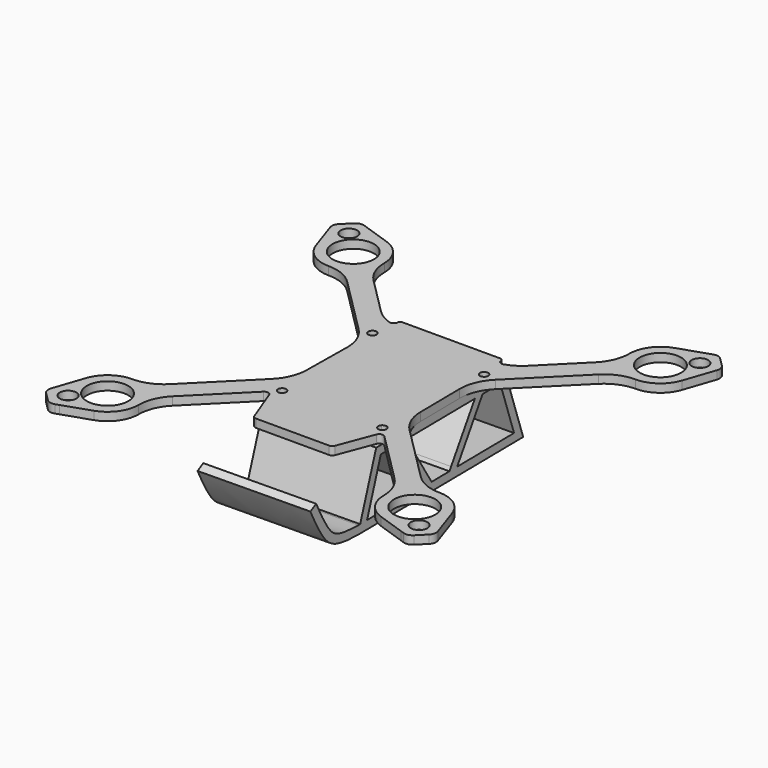
from build123d import *

# Parameters (mm, degrees)
F0_R     = 5
F0_R_2   = 1
F0_R_3   = 2
F1_DEPTH = 2
F3_DEPTH = 27


# Not quite as in the source:
# - the dataset's text gives a spline's control points without its knots; the knots are read off the source's solid


with BuildPart() as f1:
    # F0 (on Top) → F1 (new body)
    with BuildSketch(Plane.XY):
        with BuildLine():
            ThreePointArc((12.9701819491, -18.499116473), (13.6954441232, -17.876782257), (14.6119679801, -18.147501886))
            Line((14.6119679801, -18.147501886), (26.833136275, -30.3686701809))
            ThreePointArc((26.833136275, -30.3686701809), (28.8991826346, -33.4687011785), (29.6231060123, -37.1231060123))
            ThreePointArc((29.6231060123, -37.1231060123), (31.0266053165, -41.491478623), (34.7118204833, -44.2249157885))
            Line((34.7118204833, -44.2249157885), (41.2398543388, -46.4413865283))
            Line((41.2398543388, -46.4413865283), (42.1736187239, -46.7584286092))
            ThreePointArc((42.1736187239, -46.7584286092), (43.270713594, -46.8123822788), (44.2308417607, -46.2788262312))
            Line((44.2308417607, -46.2788262312), (46.2788262312, -44.2308417607))
            ThreePointArc((46.2788262312, -44.2308417607), (46.8123822788, -43.270713594), (46.7584286092, -42.1736187239))
            Line((46.7584286092, -42.1736187239), (44.2249157885, -34.7118204833))
            ThreePointArc((44.2249157885, -34.7118204833), (41.491478623, -31.0266053165), (37.1231060123, -29.6231060123))
            ThreePointArc((37.1231060123, -29.6231060123), (33.4687011785, -28.8991826346), (30.3686701809, -26.833136275))
            Line((30.3686701809, -26.833136275), (16.6740032779, -13.138469372))
            ThreePointArc((16.6740032779, -13.138469372), (14.5304846569, -9.9521662726), (13.7458594821, -6.1929691703))
            Line((13.7458594821, -6.1929691703), (13.595363536, 5.7913380039))
            ThreePointArc((13.595363536, 5.7913380039), (14.3319351196, 9.685658695), (16.5235073318, 12.9879734259))
            Line((16.5235073318, 12.9879734259), (30.3686701809, 26.833136275))
            ThreePointArc((30.3686701809, 26.833136275), (33.4687011785, 28.8991826346), (37.1231060123, 29.6231060123))
            ThreePointArc((37.1231060123, 29.6231060123), (41.491478623, 31.0266053165), (44.2249157885, 34.7118204833))
            Line((44.2249157885, 34.7118204833), (46.7584286092, 42.1736187239))
            ThreePointArc((46.7584286092, 42.1736187239), (46.8123822788, 43.270713594), (46.2788262312, 44.2308417607))
            Line((46.2788262312, 44.2308417607), (44.2308417607, 46.2788262312))
            ThreePointArc((44.2308417607, 46.2788262312), (43.270713594, 46.8123822788), (42.1736187239, 46.7584286092))
            Line((42.1736187239, 46.7584286092), (34.7118204833, 44.2249157885))
            ThreePointArc((34.7118204833, 44.2249157885), (31.0266053165, 41.491478623), (29.6231060123, 37.1231060123))
            ThreePointArc((29.6231060123, 37.1231060123), (28.8991826346, 33.4687011785), (26.833136275, 30.3686701809))
            Line((26.833136275, 30.3686701809), (17.7702922699, 21.3058261758))
            ThreePointArc((17.7702922699, 21.3058261758), (15.9339308633, 19.8564568598), (13.811079491, 18.8734020898))
            ThreePointArc((13.811079491, 18.8734020898), (12.9130317821, 19.0140644564), (12.4998939877, 19.8237512796))
            ThreePointArc((12.4998939877, 19.8237512796), (12.2538790329, 20.1992659281), (11.8415892299, 20.3768939877))
            Line((11.8415892299, 20.3768939877), (11.6629678581, 20.3768939877))
            Line((11.6629678581, 20.3768939877), (0, 20.3768939877))
            Line((0, 20.3768939877), (-11.6629678581, 20.3768939877))
            ThreePointArc((-11.6629678581, 20.3768939877), (-12.1822006328, 20.2527910691), (-12.4998939877, 19.8237512796))
            ThreePointArc((-12.4998939877, 19.8237512796), (-12.9130317821, 19.0140644564), (-13.811079491, 18.8734020898))
            ThreePointArc((-13.811079491, 18.8734020898), (-15.9339308633, 19.8564568598), (-17.7702922699, 21.3058261758))
            Line((-17.7702922699, 21.3058261758), (-26.833136275, 30.3686701809))
            ThreePointArc((-26.833136275, 30.3686701809), (-28.8991826346, 33.4687011785), (-29.6231060123, 37.1231060123))
            ThreePointArc((-29.6231060123, 37.1231060123), (-31.0266053165, 41.491478623), (-34.7118204833, 44.2249157885))
            Line((-34.7118204833, 44.2249157885), (-42.1736187239, 46.7584286092))
            ThreePointArc((-42.1736187239, 46.7584286092), (-43.270713594, 46.8123822788), (-44.2308417607, 46.2788262312))
            Line((-44.2308417607, 46.2788262312), (-46.2788262312, 44.2308417607))
            ThreePointArc((-46.2788262312, 44.2308417607), (-46.8123822788, 43.270713594), (-46.7584286092, 42.1736187239))
            Line((-46.7584286092, 42.1736187239), (-44.2249157885, 34.7118204833))
            ThreePointArc((-44.2249157885, 34.7118204833), (-41.491478623, 31.0266053165), (-37.1231060123, 29.6231060123))
            ThreePointArc((-37.1231060123, 29.6231060123), (-33.4687011785, 28.8991826346), (-30.3686701809, 26.833136275))
            Line((-30.3686701809, 26.833136275), (-16.5235073318, 12.9879734259))
            ThreePointArc((-16.5235073318, 12.9879734259), (-14.3319351196, 9.685658695), (-13.595363536, 5.7913380039))
            Line((-13.595363536, 5.7913380039), (-13.7458594821, -6.1929691703))
            ThreePointArc((-13.7458594821, -6.1929691703), (-14.5304846569, -9.9521662726), (-16.6740032779, -13.138469372))
            Line((-16.6740032779, -13.138469372), (-30.3686701809, -26.833136275))
            ThreePointArc((-30.3686701809, -26.833136275), (-33.4687011785, -28.8991826346), (-37.1231060123, -29.6231060123))
            ThreePointArc((-37.1231060123, -29.6231060123), (-41.491478623, -31.0266053165), (-44.2249157885, -34.7118204833))
            Line((-44.2249157885, -34.7118204833), (-46.7584286092, -42.1736187239))
            ThreePointArc((-46.7584286092, -42.1736187239), (-46.8123822788, -43.270713594), (-46.2788262312, -44.2308417607))
            Line((-46.2788262312, -44.2308417607), (-44.2308417607, -46.2788262312))
            ThreePointArc((-44.2308417607, -46.2788262312), (-43.270713594, -46.8123822788), (-42.1736187239, -46.7584286092))
            Line((-42.1736187239, -46.7584286092), (-41.2398543388, -46.4413865283))
            Line((-41.2398543388, -46.4413865283), (-34.7118204833, -44.2249157885))
            ThreePointArc((-34.7118204833, -44.2249157885), (-31.0266053165, -41.491478623), (-29.6231060123, -37.1231060123))
            ThreePointArc((-29.6231060123, -37.1231060123), (-28.8991826346, -33.4687011785), (-26.833136275, -30.3686701809))
            Line((-26.833136275, -30.3686701809), (-14.6119679801, -18.147501886))
            ThreePointArc((-14.6119679801, -18.147501886), (-13.6954441232, -17.876782257), (-12.9701819491, -18.499116473))
            Line((-12.9701819491, -18.499116473), (-9.7451295395, -26.9785982064))
            ThreePointArc((-9.7451295395, -26.9785982064), (-9.3781244066, -27.4463593737), (-8.8104502897, -27.6231060123))
            Line((-8.8104502897, -27.6231060123), (0, -27.6231060123))
            Line((0, -27.6231060123), (8.8104502897, -27.6231060123))
            ThreePointArc((8.8104502897, -27.6231060123), (9.3781244066, -27.4463593737), (9.7451295395, -26.9785982064))
            Line((9.7451295395, -26.9785982064), (12.9701819491, -18.499116473))
        make_face()
        with BuildLine():
            ThreePointArc((-40.4264068712, -42.4264068712), (-41.6610400065, -44.2741659362), (-43.8406204336, -43.8406204336))
            ThreePointArc((-43.8406204336, -43.8406204336), (-43.1917737359, -40.5786478062), (-40.4264068712, -42.4264068712))
        make_face(mode=Mode.SUBTRACT)
        with Locations((-37.1231060123, -37.1231060123)):
            Circle(F0_R, mode=Mode.SUBTRACT)
        with Locations((-12.1231060123, -15.6231060123)):
            Circle(F0_R_2, mode=Mode.SUBTRACT)
        with BuildLine():
            ThreePointArc((44.4264068712, -42.4264068712), (44.2741659362, -43.1917737359), (43.8406204336, -43.8406204336))
            ThreePointArc((43.8406204336, -43.8406204336), (40.5786478062, -41.6610400065), (44.4264068712, -42.4264068712))
        make_face(mode=Mode.SUBTRACT)
        with Locations((37.1231060123, -37.1231060123)):
            Circle(F0_R, mode=Mode.SUBTRACT)
        with BuildLine():
            ThreePointArc((11.398455522, -14.9339894279), (12.4941515012, -14.6944913209), (13.1231060123, -15.6231060123))
            ThreePointArc((13.1231060123, -15.6231060123), (13.0421045391, -16.0173669764), (12.8122225967, -16.3477565026))
            ThreePointArc((12.8122225967, -16.3477565026), (11.4159992311, -16.3302127935), (11.398455522, -14.9339894279))
        make_face(mode=Mode.SUBTRACT)
        with Locations((-13.4998939877, 13.3768939877)):
            Circle(F0_R_2, mode=Mode.SUBTRACT)
        with Locations((-37.1231060123, 37.1231060123)):
            Circle(F0_R, mode=Mode.SUBTRACT)
        with Locations((-42.4264068712, 42.4264068712)):
            Circle(F0_R_3, mode=Mode.SUBTRACT)
        with BuildLine():
            ThreePointArc((12.4998939877, 13.3768939877), (13.4998939877, 14.3768939877), (14.4998939877, 13.3768939877))
            ThreePointArc((14.4998939877, 13.3768939877), (13.4998939877, 12.3768939877), (12.4998939877, 13.3768939877))
        make_face(mode=Mode.SUBTRACT)
        with Locations((37.1231060123, 37.1231060123)):
            Circle(F0_R, mode=Mode.SUBTRACT)
        with Locations((42.4264068712, 42.4264068712)):
            Circle(F0_R_3, mode=Mode.SUBTRACT)
    extrude(amount=F1_DEPTH)

    # F2 (on face) → F3 (join)
    with BuildSketch(Plane(origin=(13.6659346385, 0.1716134052, 0), x_dir=(-0.012556761, 0.9999211608, 0), z_dir=(0.9999211608, 0.012556761, 0))):
        with BuildLine():
            add(Edge.make_bspline(
                [(-25.4583843052, -16.2464268506), (-25.4834532166, -16.2456672406), (-25.5084559915, -16.2448988839), (-25.5333928915, -16.2441216895)],
                knots=[0, 0, 0, 0, 0.0021421459, 0.0021421459, 0.0021421459, 0.0021421459], degree=3))
            Line((-25.4583843052, -16.2464268506), (25.1909345388, -16.2464268506))
            Line((25.1909345388, -16.2464268506), (19.5842329389, 0))
            Line((19.5842329389, 0), (5.6201676884, 0))
            Line((5.6201676884, 0), (-6.3650843938, 0))
            Line((-6.3650843938, 0), (-19.9274868111, 0))
            Line((-19.9274868111, 0), (-24.8442976991, -14.2473443619))
            Line((-24.8442976991, -14.2473443619), (-25.397810354, -14.2473443619))
            add(Edge.make_bspline(
                [(-25.397810354, -14.2473443619), (-26.82732908, -14.2040286918), (-28.6079927387, -14.0950084075), (-30.3644484255, -13.8307654603), (-31.4024158422, -13.5748028833), (-32.2061464983, -13.2672377943), (-32.8499811512, -12.9055275986), (-33.4266827552, -12.4549539511), (-33.9108707557, -11.955574038), (-34.318164566, -11.4583247593), (-34.7428114412, -10.8909327342), (-35.2912360494, -10.0734127091), (-35.9423896722, -8.9932569778), (-36.5626925571, -7.8809471841), (-37.1322447096, -6.7999448863), (-37.6335617058, -5.811017808), (-38.0524809378, -4.9695560645), (-38.2690809897, -4.5399764972), (-38.3668044786, -4.3543171965)],
                knots=[0, 0, 0, 0, 0.125, 0.1875, 0.25, 0.3125, 0.375, 0.4375, 0.5, 0.53125, 0.5625, 0.625, 0.6875, 0.75, 0.8125, 0.875, 0.9375, 1, 1, 1, 1], degree=3))
            Line((-38.3668044786, -4.3543171965), (-40.1366092265, -5.2858702838))
            add(Edge.make_bspline(
                [(-25.5333928915, -16.2441216895), (-31.7122827646, -16.0515476991), (-35.7250373114, -14.6694585794), (-39.5066402853, -6.4827124588), (-40.1366092265, -5.2858702838)],
                knots=[0.0021421459, 0.0021421459, 0.0021421459, 0.0021421459, 0.5329251902, 1, 1, 1, 1], degree=3))
        make_face()
        Polygon((-22.7282338697, -14.2464268507), (-18.5019469668, -2), (-13.0698097334, -2), (-10.6988078955, -2), (10.3555540233, -2), (12.7265558612, -2), (18.1586930968, -2), (22.3849799978, -14.2464268507), (4.9290102795, -14.2464268507), (2.5580084416, -14.2464268507), (-2.9012623138, -14.2464268507), (-5.2722641517, -14.2464268507), align=None, mode=Mode.SUBTRACT)
        Polygon((-10.6988078955, -2), (-13.0698097334, -2), (-5.2722641517, -14.2464268507), (-2.9012623138, -14.2464268507), (-3.4128590487, -13.4429391474), align=None)
        Polygon((12.7265558612, -2), (10.3555540233, -2), (3.0696051765, -13.4429391474), (2.5580084416, -14.2464268507), (4.9290102795, -14.2464268507), align=None)
    extrude(amount=-F3_DEPTH)


solid = f1.part
